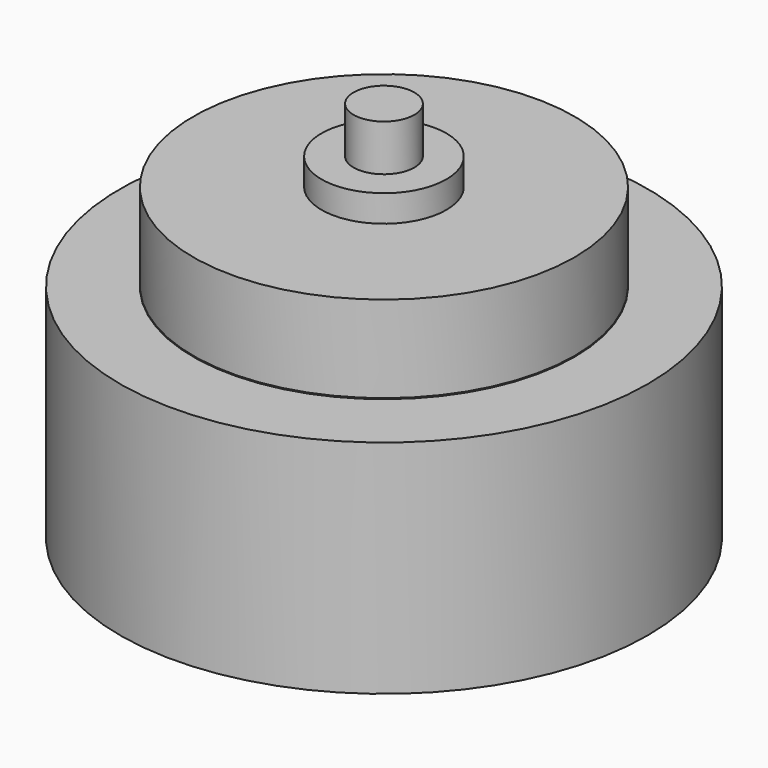
from build123d import *

# Parameters (mm, degrees)
F0_R      = 56.9
F1_DEPTH  = 47.7
F2_R      = 56.85
F3_DEPTH  = 47.6
F4_R      = 41.1
F5_DEPTH  = 66.6
F6_DEPTH  = 47.9
F7_R      = 13.45
F8_DEPTH  = 72.4
F9_DEPTH  = 66.4
F10_R     = 6.55
F11_DEPTH = 82.4
F12_DEPTH = 72.4


with BuildPart() as f1:
    # F0 (on Top) → F1 (new body)
    with BuildSketch(Plane.XY):
        Circle(F0_R)
    extrude(amount=F1_DEPTH)

    # F2 (on Top) → F3 (cut)
    with BuildSketch(Plane.XY):
        Circle(F2_R)
    extrude(amount=F3_DEPTH, mode=Mode.SUBTRACT)


with BuildPart() as f5:
    # F4 (on Top) → F5 (new body)
    with BuildSketch(Plane.XY):
        Circle(F4_R)
    extrude(amount=F5_DEPTH)


with BuildPart() as f6_tool:
    # F4 (on Top) → F6 (new body)
    with BuildSketch(Plane.XY):
        Circle(F4_R)
    extrude(amount=F6_DEPTH)


with BuildPart() as f1_1:
    add(f1.part)

    # F6: cut by f6_tool
    add(f6_tool.part, mode=Mode.SUBTRACT)


with BuildPart() as f5_1:
    add(f5.part)

    # F6: cut by f6_tool
    add(f6_tool.part, mode=Mode.SUBTRACT)


with BuildPart() as f8:
    # F7 (on Top) → F8 (new body)
    with BuildSketch(Plane.XY):
        Circle(F7_R)
    extrude(amount=F8_DEPTH)

    # F7 (on Top) → F9 (cut)
    with BuildSketch(Plane.XY):
        Circle(F7_R)
    extrude(amount=F9_DEPTH, mode=Mode.SUBTRACT)


with BuildPart() as f11:
    # F10 (on Top) → F11 (new body)
    with BuildSketch(Plane.XY):
        Circle(F10_R)
    extrude(amount=F11_DEPTH)

    # F10 (on Top) → F12 (cut)
    with BuildSketch(Plane.XY):
        Circle(F10_R)
    extrude(amount=F12_DEPTH, mode=Mode.SUBTRACT)


solid = Compound([f1_1.part, f5_1.part, f8.part, f11.part])
